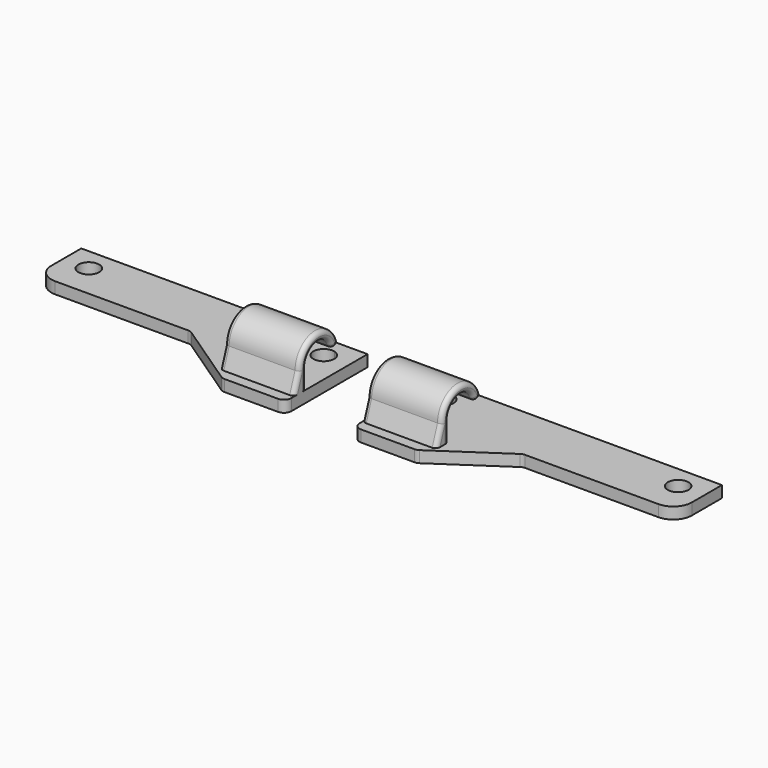
from build123d import *

# Parameters (mm, degrees)
F0_R      = 2.8
F1_DEPTH  = 3.1
F2_W      = 20
F2_H      = 2.3
F3_DEPTH  = 5.1
F3_FACE_W = 20
F3_FACE_H = 2.3
F5_ANGLE  = 170
F6_R      = 1.14999
F8_DEPTH  = 20
F9_R      = 1.14


# Not quite as in the source:
# - a fillet or chamfer is up to 0.001 mm smaller than in the source, because OpenCascade refuses the exact size


with BuildPart() as f1:
    # F0 (on Top) → F1 (new body)
    with BuildSketch(Plane.XY):
        with BuildLine():
            Line((36.738385576, 27.4999964178), (-29.061614424, 27.4999964178))
            Line((-29.061614424, 27.4999964178), (-34.061614424, 27.4999964178))
            Line((-34.061614424, 27.4999964178), (-34.061614424, 22.4999964178))
            Line((-34.061614424, 22.4999964178), (-34.061614424, 17.3999964178))
            ThreePointArc((-34.061614424, 17.3999964178), (-32.5971483299, 13.8644625118), (-29.061614424, 12.3999964178))
            Line((-29.061614424, 12.3999964178), (6.7794218737, 12.3999964178))
            ThreePointArc((6.7794218737, 12.3999964178), (7.3637845142, 12.312722301), (7.8971474214, 12.0585167222))
            Line((7.8971474214, 12.0585167222), (25.4316860469, 0.2414761133))
            ThreePointArc((25.4316860469, 0.2414761133), (25.9650489541, -0.0127294655), (26.5494115945, -0.1000035822))
            Line((26.5494115945, -0.1000035822), (40.938385576, -0.1000035822))
            ThreePointArc((40.938385576, -0.1000035822), (42.3525991384, 0.4857828554), (42.938385576, 1.8999964178))
            Line((42.938385576, 1.8999964178), (42.938385576, 12.3999964178))
            Line((42.938385576, 12.3999964178), (42.938385576, 22.4999964178))
            Line((42.938385576, 22.4999964178), (42.938385576, 27.4999964178))
            Line((42.938385576, 27.4999964178), (37.938385576, 27.4999964178))
            Line((37.938385576, 27.4999964178), (36.738385576, 27.4999964178))
        make_face()
        with Locations((-27.161614424, 21.3999964178)):
            Circle(F0_R, mode=Mode.SUBTRACT)
        with BuildLine():
            ThreePointArc((38.838385576, 21.3999964178), (33.8247912139, 19.6853535978), (36.738385576, 24.1110847601))
            ThreePointArc((36.738385576, 24.1110847601), (38.2519799381, 23.1146392377), (38.838385576, 21.3999964178))
        make_face(mode=Mode.SUBTRACT)
    extrude(amount=F1_DEPTH)

    # F2 (on face) → F3 (join)
    with BuildSketch(Plane.XY.offset(3.1)):
        with Locations((32.938385576, 5.6874617912)):
            Rectangle(F2_W, F2_H)
    extrude(amount=F3_DEPTH)

    # F3_face (on face) → F5 (revolve)
    with BuildSketch(Plane(origin=(32.938385576, 5.6874617912, 8.2), x_dir=(1, 0, 0), z_dir=(0, 0, 1))):
        Rectangle(F3_FACE_W, F3_FACE_H)
    revolve(axis=Axis((32.938385576, 11.2540264437, 8.2), (-1, 0, 0)), revolution_arc=F5_ANGLE)

    # F6 (radius 1.15 in the source; OpenCascade refuses exactly that, so slightly less here)
    f6_edges = [f1.edges().sort_by_distance(p)[0] for p in [
        (32.938386, 15.603494, 8.966928),
        (32.938386, 17.868551, 9.366319),
    ]]
    fillet(f6_edges, radius=F6_R)

    # F7 (on face) → F8 (join)
    with BuildSketch(Plane(origin=(22.938385576, 0, 0), x_dir=(0, -1, 0), z_dir=(-1, 0, 0))):
        Polygon((-2.7374617912, 3.1), (-4.5374617912, 8.2), (-4.5374617912, 3.1), align=None)
    extrude(amount=-F8_DEPTH)

    # F9
    f9_edges = [f1.edges().sort_by_distance(p)[0] for p in [
        (22.938386, 3.637462, 5.65),
        (22.938386, 9.976905, 14.794028),
        (42.938386, 3.637462, 5.65),
        (42.938386, 9.976905, 14.794028),
    ]]
    fillet(f9_edges, radius=F9_R)


with BuildPart() as f1_1:
    # F10: moved
    add(f1.part.moved(Location((-52.1, 0, 0))))


with BuildPart() as f11_1:
    # F11: instance of F1
    add(f1_1.part.mirror(Plane.YZ))


solid = Compound([f1_1.part, f11_1.part])
